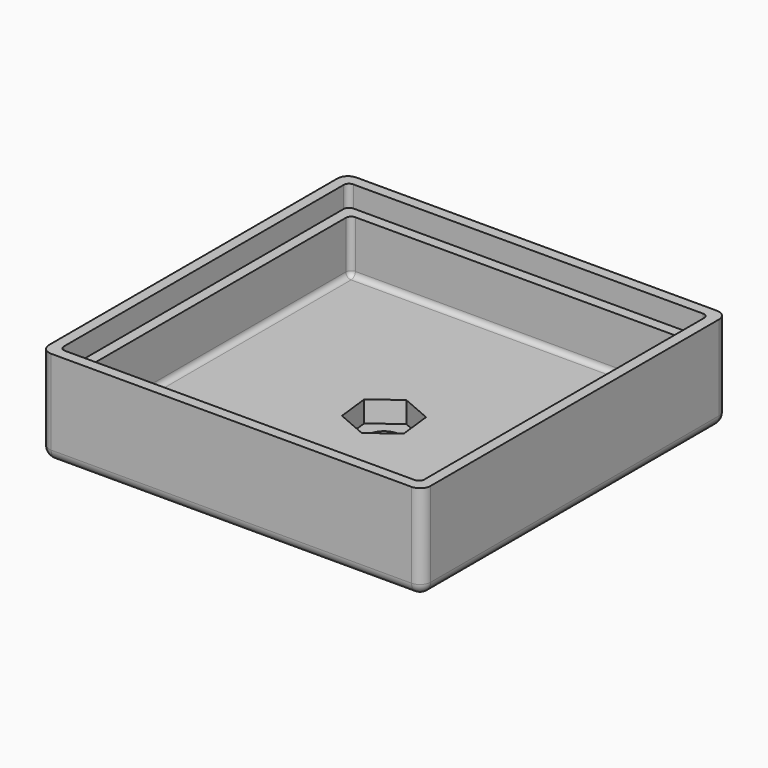
from build123d import *

# Parameters (mm, degrees)
F1_W         = 36
F1_H         = 36
F2_DEPTH     = 9
F3_T         = -2
F4_START     = 7
F0_W         = 34
F0_H         = 34
F4_DEPTH     = 3
F5_R         = 1
F6_R         = 0.5
F7_T1_DEPTH  = 10.5
F7_S5_W      = 1
F7_S5_H      = 1
F7_T6_DEPTH  = 1
F7_S11_W     = 1
F7_S11_H     = 1
F7_T12_DEPTH = 1
F7_S17_W     = 1
F7_S17_H     = 1
F7_T18_DEPTH = 1
F7_S23_W     = 1
F7_S23_H     = 1
F7_T24_DEPTH = 1
F9_DEPTH     = 2
F11_START    = -1.5
F10_W        = 12.2
F10_H        = 20.1
F11_DEPTH    = 2.5
F13_DEPTH    = 2
F14_R        = 1.5
F15_DEPTH    = 4.001
F16_R        = 0.5
F17_R        = 0.5


# Not quite as in the source:
# - a fillet or chamfer that OpenCascade refuses, or shapes differently, is made with other operations: its cross-section is extruded or revolved along the edge and cut away or added


with BuildPart() as f2:
    # F1 (on Top) → F2 (new body)
    with BuildSketch(Plane.XY):
        Rectangle(F1_W, F1_H)
    extrude(amount=F2_DEPTH)

    # F3
    f3_openings = [f2.faces().sort_by_distance(p)[0] for p in [
        (0, 0, 9),
    ]]
    offset(amount=F3_T, openings=f3_openings)

    # F0 (on Top) → F4 (cut)
    with BuildSketch(Plane.XY.offset(F4_START)):
        Rectangle(F0_W, F0_H)
    extrude(amount=F4_DEPTH, mode=Mode.SUBTRACT)

    # F5
    f5_edges = [f2.edges().sort_by_distance(p)[0] for p in [
        (18, 0, 0),
        (0, 18, 0),
        (-18, 0, 0),
        (0, -18, 0),
    ]]
    fillet(f5_edges, radius=F5_R)

    # F6
    f6_edges = [f2.edges().sort_by_distance(p)[0] for p in [
        (0, 16, 2),
        (-16, 0, 2),
        (0, -16, 2),
        (16, 0, 2),
        (-16, 16, 4.5),
        (16, 16, 4.5),
        (17, 17, 8),
        (17, -17, 8),
        (16, -16, 4.5),
        (-17, -17, 8),
        (-16, -16, 4.5),
        (-17, 17, 8),
    ]]
    fillet(f6_edges, radius=F6_R)

    # F7: fillet of radius 1 on 4 edges, made by hand

    # F7_s2 → F7_t1 (cut)
    with BuildSketch(Plane.XY.offset(1)):
        with BuildLine():
            ThreePointArc((-18, -17), (-17.7071067812, -17.7071067812), (-17, -18))
            Line((-17, -18), (-18, -18))
            Line((-18, -18), (-18, -17))
        make_face()
        with BuildLine():
            ThreePointArc((17, 18), (17.7071067812, 17.7071067812), (18, 17))
            Line((18, 17), (18, 18))
            Line((18, 18), (17, 18))
        make_face()
        with BuildLine():
            ThreePointArc((18, -17), (17.7071067812, -17.7071067812), (17, -18))
            Line((17, -18), (18, -18))
            Line((18, -18), (18, -17))
        make_face()
        with BuildLine():
            ThreePointArc((-17, 18), (-17.7071067812, 17.7071067812), (-18, 17))
            Line((-18, 17), (-18, 18))
            Line((-18, 18), (-17, 18))
        make_face()
    extrude(amount=F7_T1_DEPTH, mode=Mode.SUBTRACT)


with BuildPart() as f7_tool4:
    # F7_s5 → F7_t6 (new body)
    with BuildSketch(Plane.XZ.offset(-17)):
        with Locations((-17.5, 0.5)):
            Rectangle(F7_S5_W, F7_S5_H)
    extrude(amount=-F7_T6_DEPTH)

    # F7_s7 → F7_t8 (revolve, cut)
    with BuildSketch(Plane(origin=(-17, 17, 1), x_dir=(0.7071067812, 0, 0.7071067812), z_dir=(-0.7071067812, 0, 0.7071067812))):
        with BuildLine():
            ThreePointArc((0, -1), (1, 0), (0, 1))
            Line((0, 1), (0, -1))
        make_face()
    revolve(axis=Axis((-17, 17, 1), (0, 1, 0)), mode=Mode.SUBTRACT)


with BuildPart() as f2_1:
    add(f2.part)

    # F7_t3: cut F7_tool4
    add(f7_tool4.part, mode=Mode.SUBTRACT)


with BuildPart() as f7_tool10:
    # F7_s11 → F7_t12 (new body)
    with BuildSketch(Plane.YZ.offset(17)):
        with Locations((-17.5, 0.5)):
            Rectangle(F7_S11_W, F7_S11_H)
    extrude(amount=F7_T12_DEPTH)

    # F7_s13 → F7_t14 (revolve, cut)
    with BuildSketch(Plane(origin=(17, -17, 1), x_dir=(0, 0.7071067812, 0.7071067812), z_dir=(0, 0.7071067812, -0.7071067812))):
        with BuildLine():
            ThreePointArc((0, -1), (1, 0), (0, 1))
            Line((0, 1), (0, -1))
        make_face()
    revolve(axis=Axis((17, -17, 1), (1, 0, 0)), mode=Mode.SUBTRACT)


with BuildPart() as f2_2:
    add(f2_1.part)

    # F7_t9: cut F7_tool10
    add(f7_tool10.part, mode=Mode.SUBTRACT)


with BuildPart() as f7_tool16:
    # F7_s17 → F7_t18 (new body)
    with BuildSketch(Plane.XZ.offset(-17)):
        with Locations((17.5, 0.5)):
            Rectangle(F7_S17_W, F7_S17_H)
    extrude(amount=-F7_T18_DEPTH)

    # F7_s19 → F7_t20 (revolve, cut)
    with BuildSketch(Plane(origin=(17, 17, 1), x_dir=(-0.7071067812, 0, 0.7071067812), z_dir=(-0.7071067812, 0, -0.7071067812))):
        with BuildLine():
            ThreePointArc((0, -1), (1, 0), (0, 1))
            Line((0, 1), (0, -1))
        make_face()
    revolve(axis=Axis((17, 17, 1), (0, 1, 0)), mode=Mode.SUBTRACT)


with BuildPart() as f2_3:
    add(f2_2.part)

    # F7_t15: cut F7_tool16
    add(f7_tool16.part, mode=Mode.SUBTRACT)


with BuildPart() as f7_tool22:
    # F7_s23 → F7_t24 (new body)
    with BuildSketch(Plane.YZ.offset(-17)):
        with Locations((-17.5, 0.5)):
            Rectangle(F7_S23_W, F7_S23_H)
    extrude(amount=-F7_T24_DEPTH)

    # F7_s25 → F7_t26 (revolve, cut)
    with BuildSketch(Plane(origin=(-17, -17, 1), x_dir=(0, 0.7071067812, 0.7071067812), z_dir=(0, -0.7071067812, 0.7071067812))):
        with BuildLine():
            ThreePointArc((0, -1), (1, 0), (0, 1))
            Line((0, 1), (0, -1))
        make_face()
    revolve(axis=Axis((-17, -17, 1), (-1, 0, 0)), mode=Mode.SUBTRACT)


with BuildPart() as f2_4:
    add(f2_3.part)

    # F7_t21: cut F7_tool22
    add(f7_tool22.part, mode=Mode.SUBTRACT)

    # F8 (on Top) → F9 (join)
    with BuildSketch(Plane.XY):
        with BuildLine():
            ThreePointArc((-11, -11), (-10.4142135624, -12.4142135624), (-9, -13))
            Line((-9, -13), (9, -13))
            ThreePointArc((9, -13), (10.4142135624, -12.4142135624), (11, -11))
            Line((11, -11), (11, 7))
            ThreePointArc((11, 7), (9.5355339059, 10.5355339059), (6, 12))
            Line((6, 12), (-6, 12))
            ThreePointArc((-6, 12), (-9.5355339059, 10.5355339059), (-11, 7))
            Line((-11, 7), (-11, -11))
        make_face()
    extrude(amount=-F9_DEPTH)

    # F10 (on Top) → F11 (cut)
    with BuildSketch(Plane.XY.offset(F11_START)):
        with Locations((0, -2.95)):
            Rectangle(F10_W, F10_H)
    extrude(amount=-F11_DEPTH, mode=Mode.SUBTRACT)

    # F12 (on face) → F13 (cut)
    with BuildSketch(Plane.XY.offset(2)):
        Polygon((-0.3596221451, 3.0790699753), (-2.8463638912, 1.2280930742), (-2.4867417461, -1.850976901), (0.3596221451, -3.0790699753), (2.8463638912, -1.2280930742), (2.4867417461, 1.850976901), align=None)
    extrude(amount=-F13_DEPTH, mode=Mode.SUBTRACT)

    # F14 (on face) → F15 (cut, through all)
    with BuildSketch(Plane.XY.offset(2)):
        Circle(F14_R)
    extrude(amount=-F15_DEPTH, mode=Mode.SUBTRACT)

    # F16
    f16_edges = [f2_4.edges().sort_by_distance(p)[0] for p in [
        (11, -2, 0),
        (6.1, 7.1, -1.75),
        (-6.1, 7.1, -1.75),
    ]]
    fillet(f16_edges, radius=F16_R)

    # F17
    f17_edges = [f2_4.edges().sort_by_distance(p)[0] for p in [
        (7.55, -13, -2),
    ]]
    fillet(f17_edges, radius=F17_R)


solid = f2_4.part
